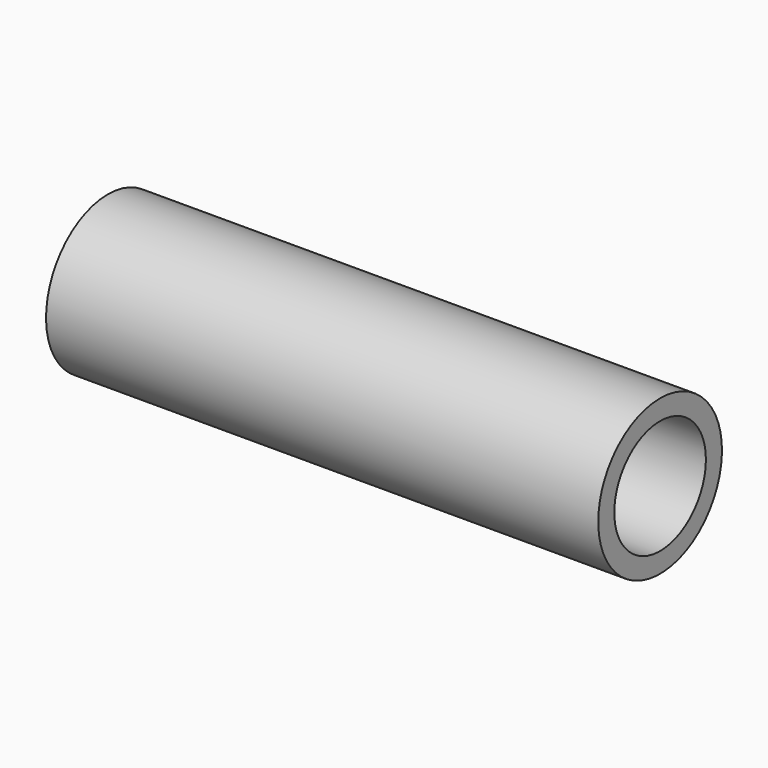
from build123d import *

# Parameters (mm, degrees)
F0_W     = 76.2
F0_H     = 10.668
F2_R     = 7.8994
F3_DEPTH = 76.2


# Not quite as in the source:
# - a feature names something its author has since deleted; it is built from what else it names


with BuildPart() as f1:
    # F0 (on Front) → F1 (revolve)
    with BuildSketch(Plane.XZ):
        with Locations((38.1, 5.334)):
            Rectangle(F0_W, F0_H)
    revolve(axis=Axis((38.1, 0, 0), (1, 0, 0)))

    # F2 (on face) → F3 (cut, through all)
    with BuildSketch(Plane.YZ.offset(76.2)):
        Circle(F2_R)
    extrude(amount=-F3_DEPTH, mode=Mode.SUBTRACT)


solid = f1.part
